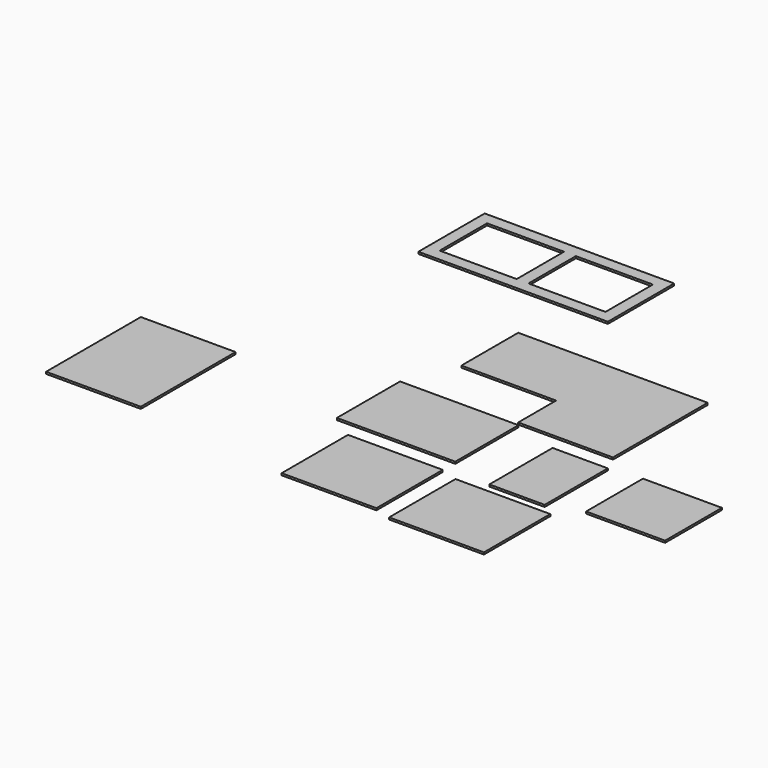
from build123d import *

# Parameters (mm, degrees)
F1_DEPTH = 12.7
F0_W     = 762
F0_H     = 508
F0_W_2   = 609.6
F0_H_2   = 533.4
F0_W_3   = 355.6
F0_W_4   = 508
F0_H_3   = 457.2
F0_H_4   = 762
F0_W_5   = 1219.2
F0_W_6   = 495.3
F0_H_5   = 381


# Not quite as in the source:
# - a feature names something its author has since deleted; it is built from what else it names


with BuildPart() as f1:
    # F0 (on Top) → F1 (new body)
    with BuildSketch(Plane.XY):
        Polygon((536.5461329095, 340.8599793494), (-682.6538670905, 340.8599793494), (-682.6538670905, -116.3400206506), (-73.0538670905, -116.3400206506), (-73.0538670905, -421.1400206506), (536.5461329095, -421.1400206506), align=None)
    extrude(amount=F1_DEPTH)


with BuildPart() as f1b:
    # F0 (on Top) → F1, piece 2 (new body)
    with BuildSketch(Plane.XY):
        with Locations((-434.3071403503, -697.7123699188)):
            Rectangle(F0_W, F0_H)
    extrude(amount=F1_DEPTH)


with BuildPart() as f1c:
    # F0 (on Top) → F1, piece 3 (new body)
    with BuildSketch(Plane.XY):
        with Locations((-351.5841700554, -1327.6137407303)):
            Rectangle(F0_W_2, F0_H_2)
    extrude(amount=F1_DEPTH)


with BuildPart() as f1d:
    # F0 (on Top) → F1, piece 4 (new body)
    with BuildSketch(Plane.XY):
        with Locations((370.4786859035, -1365.6170661926)):
            Rectangle(F0_W_2, F0_H_2)
    extrude(amount=F1_DEPTH)


with BuildPart() as f1e:
    # F0 (on Top) → F1, piece 5 (new body)
    with BuildSketch(Plane.XY):
        with Locations((412.7661439657, -784.0835533142)):
            Rectangle(F0_W_3, F0_H)
    extrude(amount=F1_DEPTH)


with BuildPart() as f1f:
    # F0 (on Top) → F1, piece 6 (new body)
    with BuildSketch(Plane.XY):
        with Locations((1052.3282208443, -735.7748402596)):
            Rectangle(F0_W_4, F0_H_3)
    extrude(amount=F1_DEPTH)


with BuildPart() as f1g:
    # F0 (on Top) → F1, piece 7 (new body)
    with BuildSketch(Plane.XY):
        with Locations((-1965.0879241943, -1091.020983696)):
            Rectangle(F0_W_2, F0_H_4)
    extrude(amount=F1_DEPTH)


with BuildPart() as f1h:
    # F0 (on Top) → F1, piece 8 (new body)
    with BuildSketch(Plane.XY):
        with Locations((-1015.4649690628, 982.4869935036)):
            Rectangle(F0_W_5, F0_H_2)
        with Locations((-1301.2149690628, 982.4869935036)):
            Rectangle(F0_W_6, F0_H_5, mode=Mode.SUBTRACT)
        with Locations((-729.7149690628, 982.4869935036)):
            Rectangle(F0_W_6, F0_H_5, mode=Mode.SUBTRACT)
    extrude(amount=F1_DEPTH)


solid = Compound([f1.part, f1b.part, f1c.part, f1d.part, f1e.part, f1f.part, f1g.part, f1h.part])
